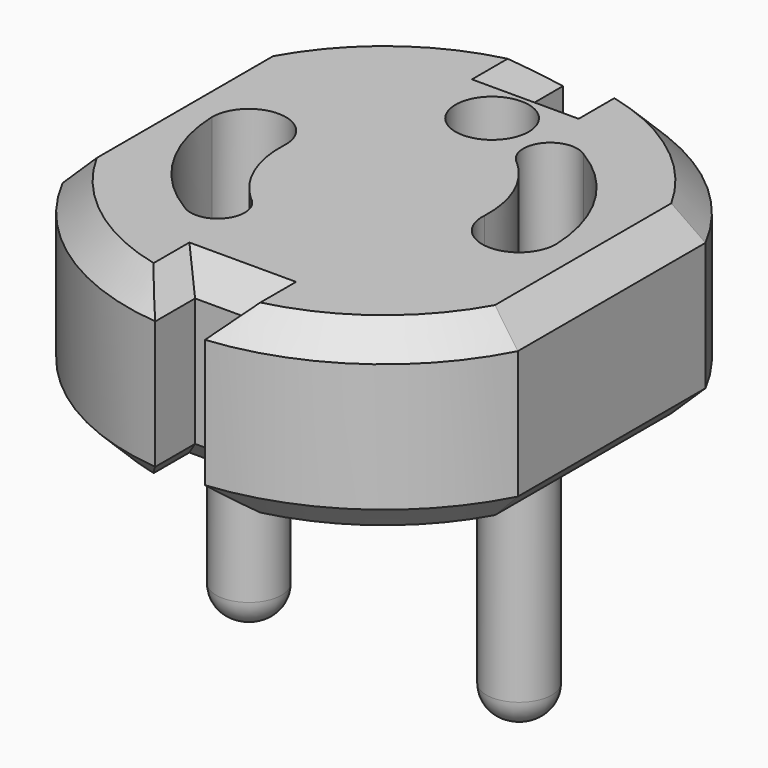
from build123d import *

# Parameters (mm, degrees)
F0_R     = 2.575
F1_DEPTH = 13
F0_R_2   = 2.3
F2_DEPTH = 3
F3_DEPTH = 17
F4_R     = 2
F5_SIZE  = 1.99999
F6_SIZE  = 1.99999


# Not quite as in the source:
# - a fillet or chamfer is up to 0.001 mm smaller than in the source, because OpenCascade refuses the exact size


with BuildPart() as f1:
    # F0 (on Top) → F1 (new body)
    with BuildSketch(Plane.XY):
        with BuildLine():
            Line((1.75, -14.4147285773), (1.75, -17.9147285773))
            ThreePointArc((1.75, -17.9147285773), (10.1062199571, -14.895110546), (16, -8.2462112512))
            Line((16, -8.2462112512), (16, 8.2462112512))
            ThreePointArc((16, 8.2462112512), (10.1062199571, 14.895110546), (1.75, 17.9147285773))
            Line((1.75, 17.9147285773), (1.75, 14.4147285773))
            Line((1.75, 14.4147285773), (-1.75, 14.4147285773))
            Line((-1.75, 14.4147285773), (-1.75, 17.9147285773))
            ThreePointArc((-1.75, 17.9147285773), (-10.1062199571, 14.895110546), (-16, 8.2462112512))
            Line((-16, 8.2462112512), (-16, -8.2462112512))
            ThreePointArc((-16, -8.2462112512), (-10.1062199571, -14.895110546), (-1.75, -17.9147285773))
            Line((-1.75, -17.9147285773), (-1.75, -14.4147285773))
            Line((-1.75, -14.4147285773), (1.75, -14.4147285773))
        make_face()
        with BuildLine():
            ThreePointArc((-12.1, 0), (-9.4098118123, 2.5984353159), (-6.9062568532, -0.1802678246))
            ThreePointArc((-6.9062568532, -0.1802678246), (-6.3236870302, -3.4718300474), (-4.3937995375, -6.2011713107))
            ThreePointArc((-4.3937995375, -6.2011713107), (-3.9419565942, -8.8499140227), (-6.5906993063, -9.301756966))
            ThreePointArc((-6.5906993063, -9.301756966), (-10.5283348632, -5.3515440951), (-12.1, 0))
        make_face(mode=Mode.SUBTRACT)
        with BuildLine():
            ThreePointArc((12.1, 0), (9.4098118123, -2.5984353159), (6.9062568532, 0.1802678246))
            ThreePointArc((6.9062568532, 0.1802678246), (6.3236870302, 3.4718300474), (4.3937995375, 6.2011713107))
            ThreePointArc((4.3937995375, 6.2011713107), (3.9419565942, 8.8499140227), (6.5906993063, 9.301756966))
            ThreePointArc((6.5906993063, 9.301756966), (10.5283348632, 5.3515440951), (12.1, 0))
        make_face(mode=Mode.SUBTRACT)
        with Locations((0, 9.5)):
            Circle(F0_R, mode=Mode.SUBTRACT)
    extrude(amount=F1_DEPTH)

    # F0 (on Top) → F2 (join)
    with BuildSketch(Plane.XY):
        with BuildLine():
            ThreePointArc((-4.3937995375, -6.2011713107), (-6.3236870302, -3.4718300474), (-6.9062568532, -0.1802678246))
            ThreePointArc((-6.9062568532, -0.1802678246), (-9.4098118123, 2.5984353159), (-12.1, 0))
            ThreePointArc((-12.1, 0), (-10.5283348632, -5.3515440951), (-6.5906993063, -9.301756966))
            ThreePointArc((-6.5906993063, -9.301756966), (-3.9419565942, -8.8499140227), (-4.3937995375, -6.2011713107))
        make_face()
        with Locations((-9.5, 0)):
            Circle(F0_R_2, mode=Mode.SUBTRACT)
        with Locations((-9.5, 0)):
            Circle(F0_R_2)
        with BuildLine():
            ThreePointArc((4.3937995375, 6.2011713107), (6.3236870302, 3.4718300474), (6.9062568532, 0.1802678246))
            ThreePointArc((6.9062568532, 0.1802678246), (9.4098118123, -2.5984353159), (12.1, 0))
            ThreePointArc((12.1, 0), (10.5283348632, 5.3515440951), (6.5906993063, 9.301756966))
            ThreePointArc((6.5906993063, 9.301756966), (3.9419565942, 8.8499140227), (4.3937995375, 6.2011713107))
        make_face()
        with Locations((9.5, 0)):
            Circle(F0_R_2, mode=Mode.SUBTRACT)
        with Locations((9.5, 0)):
            Circle(F0_R_2)
    extrude(amount=F2_DEPTH)

    # F0 (on Top) → F3 (join)
    with BuildSketch(Plane.XY):
        with Locations((-9.5, 0)):
            Circle(F0_R_2)
        with Locations((9.5, 0)):
            Circle(F0_R_2)
    extrude(amount=-F3_DEPTH)

    # F4
    f4_edges = [f1.edges().sort_by_distance(p)[0] for p in [
        (-11.8, 0, -17),
        (7.2, 0, -17),
    ]]
    fillet(f4_edges, radius=F4_R)

    # F5 (size 2 in the source; OpenCascade refuses exactly that, so slightly less here)
    f5_edges = [f1.edges().sort_by_distance(p)[0] for p in [
        (10.10622, 14.895111, 13),
        (16, 0, 13),
        (10.10622, -14.895111, 13),
        (1.75, -16.164729, 13),
        (0, -14.414729, 13),
        (-1.75, -16.164729, 13),
        (-10.10622, -14.895111, 13),
        (-16, 0, 13),
        (-10.10622, 14.895111, 13),
        (-1.75, 16.164729, 13),
        (0, 14.414729, 13),
        (1.75, 16.164729, 13),
    ]]
    chamfer(f5_edges, length=F5_SIZE)

    # F6 (size 2 in the source; OpenCascade refuses exactly that, so slightly less here)
    f6_edges = [f1.edges().sort_by_distance(p)[0] for p in [
        (10.10622, 14.895111, 0),
        (16, 0, 0),
        (10.10622, -14.895111, 0),
        (0, 14.414729, 0),
        (1.75, 16.164729, 0),
        (-1.75, 16.164729, 0),
        (-10.10622, 14.895111, 0),
        (-16, 0, 0),
        (-10.10622, -14.895111, 0),
        (-1.75, -16.164729, 0),
        (0, -14.414729, 0),
        (1.75, -16.164729, 0),
    ]]
    chamfer(f6_edges, length=F6_SIZE)


solid = f1.part
